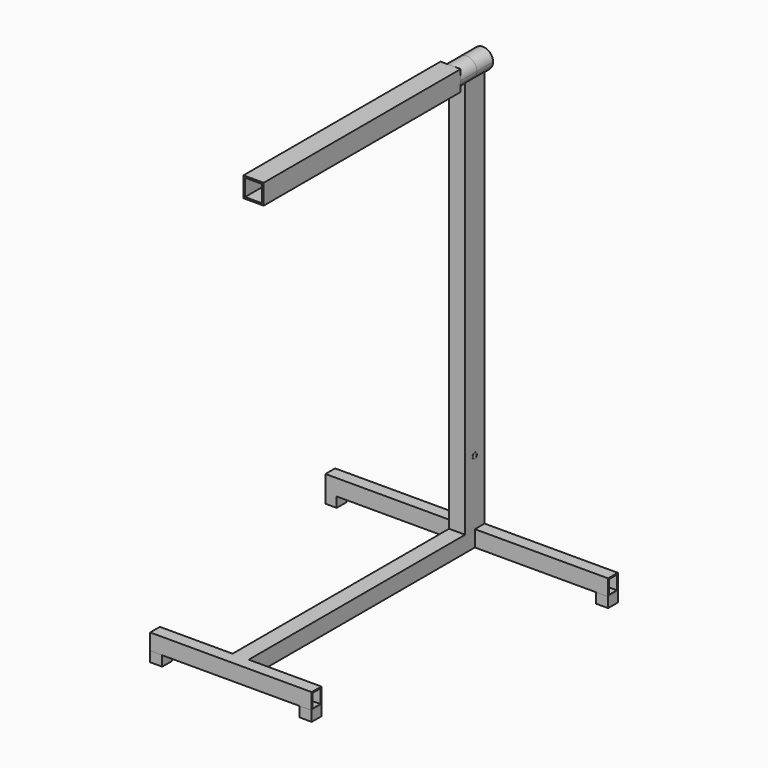
from build123d import *

# Parameters (mm, degrees)
F0_R      = 20
F1_DEPTH  = 50
F2_DEPTH  = 30
F3_W      = 32
F3_H      = 52
F4_DEPTH  = 988.001
F5_W      = 30
F5_H      = 40
F5_W_2    = 24
F5_H_2    = 34
F6_DEPTH  = 350
F8_DEPTH  = 700
F9_DEPTH  = 200
F10_W     = 27.8917610645
F10_H     = 30
F10_W_2   = 29.6796619892
F10_W_3   = 29.7341316938
F10_W_4   = 29.711586237
F11_DEPTH = 25
F12_W     = 50
F12_H     = 50
F13_DEPTH = 10
F14_W     = 50
F14_H     = 50
F14_W_2   = 42
F14_H_2   = 42
F15_DEPTH = 600
F16_R     = 7.5
F16_R_2   = 5.5
F17_DEPTH = 20.5


# Not quite as in the source:
# - the program builds the solid bodies; features that only make, move or delete a surface that nothing else refers to are left out


with BuildPart() as f1:
    # F0 (on Front) → F1 (new body, symmetric)
    with BuildSketch(Plane.XZ):
        with BuildLine():
            ThreePointArc((20, -15), (23.7170824513, -7.9056941504), (25, 0))
            ThreePointArc((25, 0), (-7.9056941504, 23.7170824513), (-20, -15))
            ThreePointArc((-20, -15), (0, -25), (20, -15))
        make_face()
        Circle(F0_R, mode=Mode.SUBTRACT)
    extrude(amount=F1_DEPTH, both=True)

    # F0 (on Front) → F2 (join, symmetric)
    with BuildSketch(Plane.XZ):
        with BuildLine():
            ThreePointArc((20, -15), (0, -25), (-20, -15))
            Line((-20, -15), (-20, -1000))
            Line((-20, -1000), (20, -1000))
            Line((20, -1000), (20, -15))
        make_face()
    extrude(amount=F2_DEPTH, both=True)

    # F3 (on face) → F4 (cut, through all)
    with BuildSketch(Plane(origin=(0, 0, -1000), x_dir=(1, 0, 0), z_dir=(0, 0, -1))):
        Rectangle(F3_W, F3_H)
    extrude(amount=-F4_DEPTH, mode=Mode.SUBTRACT)

    # F5 (on Right) → F6 (join, symmetric)
    with BuildSketch(Plane.YZ):
        with Locations((15, -1020)):
            Rectangle(F5_W, F5_H)
        with Locations((15, -1020)):
            Rectangle(F5_W_2, F5_H_2, mode=Mode.SUBTRACT)
    extrude(amount=F6_DEPTH, both=True)

    # F7 (on face) → F8 (join)
    with BuildSketch(Plane.XZ):
        Polygon((-16, -1000), (-20, -1000), (-20, -1020), (-20, -1040), (20, -1040), (20, -1000), (16, -1000), align=None)
        Polygon((-17, -1037), (-17, -1020), (-17, -1003), (17, -1003), (17, -1037), align=None, mode=Mode.SUBTRACT)
    extrude(amount=F8_DEPTH)

    # F5 (on Right) → F9 (join, symmetric)
    with BuildSketch(Plane.YZ):
        with Locations((-715, -1020)):
            Rectangle(F5_W, F5_H)
        with Locations((-715, -1020)):
            Rectangle(F5_W_2, F5_H_2, mode=Mode.SUBTRACT)
    extrude(amount=F9_DEPTH, both=True)

    # F10 (on face) → F11 (join)
    with BuildSketch(Plane(origin=(0, 0, -1040), x_dir=(1, 0, 0), z_dir=(0, 0, -1))):
        with Locations((-336.0541194677, -15)):
            Rectangle(F10_W, F10_H)
        with Locations((335.1601690054, -15)):
            Rectangle(F10_W_2, F10_H)
        with Locations((-185.1329341531, 715)):
            Rectangle(F10_W_3, F10_H)
        with Locations((185.1442068815, 715)):
            Rectangle(F10_W_4, F10_H)
    extrude(amount=F11_DEPTH)

    # F12 (on face) → F13 (join)
    with BuildSketch(Plane.XZ.offset(50)):
        Rectangle(F12_W, F12_H)
    extrude(amount=F13_DEPTH)

    # F14 (on face) → F15 (join)
    with BuildSketch(Plane.XZ.offset(60)):
        Rectangle(F14_W, F14_H)
        Rectangle(F14_W_2, F14_H_2, mode=Mode.SUBTRACT)
    extrude(amount=F15_DEPTH)

    # F16 (on Right) → F17 (join, symmetric)
    with BuildSketch(Plane.YZ):
        with Locations((0, -840)):
            Circle(F16_R)
        with Locations((0, -840)):
            Circle(F16_R_2, mode=Mode.SUBTRACT)
    extrude(amount=F17_DEPTH, both=True)


solid = f1.part
